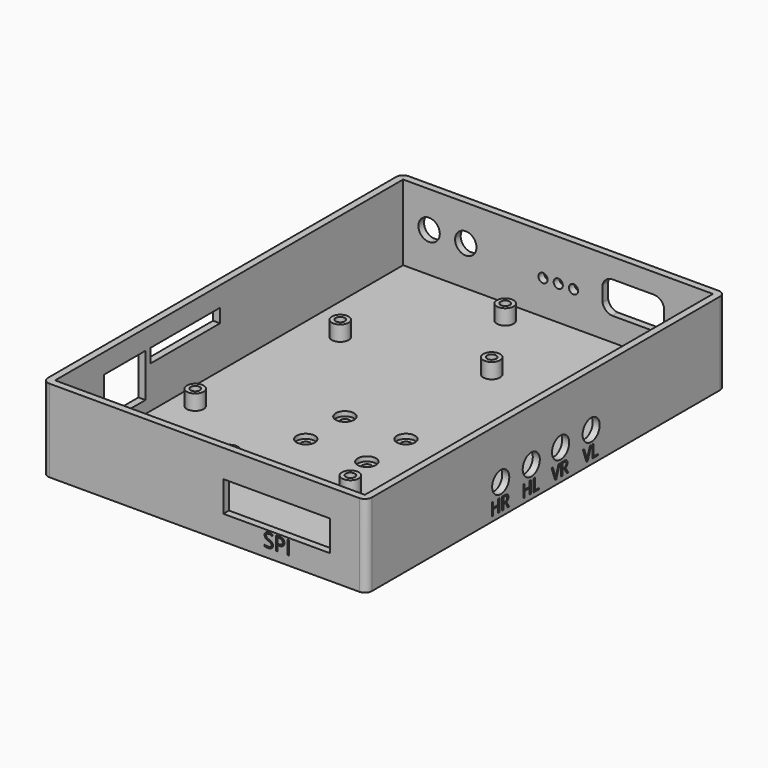
from build123d import *

# Parameters (mm, degrees)
F0_W            = 106
F0_H            = 147
F1_DEPTH        = 27
F2_T            = -2.3
F3_W            = 17
F3_H            = 14.2
F3_W_2          = 28.5
F3_H_2          = 4.5
F4_DEPTH        = 2.3
F5_R            = 2.3
F7_DEPTH        = 2.3
F9_DEPTH        = 2.3
F10_R           = 3.5
F10_R_2         = 1.5
F11_DEPTH       = 2.3
F12_TEXT_SIZE   = 5.6944444444
F13_DEPTH       = 1.0021
F14_TEXT_SIZE   = 6.25
F15_DEPTH       = 1
F16_TEXT_SIZE   = 4.2000262502
F16_TEXT_SIZE_2 = 6.8394336094
F16_TEXT_SIZE_3 = 6.6666666667
F16_TEXT_SIZE_4 = 6.25
F17_DEPTH       = 1
F18_DEPTH       = 1
F20_R           = 3
F20_R_2         = 1.5
F21_DEPTH       = 1.5
F22_DEPTH       = 2.3
F23_R           = 2.75
F24_DEPTH       = 5
F25_R           = 1.527073586
F26_DEPTH       = 2.5
F27_R           = 1.5414373887
F28_DEPTH       = 2.5
F29_R           = 1.5334502913
F30_DEPTH       = 2.5
F31_R           = 1.5249444559
F32_DEPTH       = 2.5
F33_R           = 1.5
F34_DEPTH       = 2.5
F35_R           = 1.5
F36_DEPTH       = 2.5
F37_R           = 1.5
F38_DEPTH       = 5
F39_R           = 1.5
F40_DEPTH       = 5
F41_R           = 1.5
F42_DEPTH       = 5
F43_R           = 1.5
F44_DEPTH       = 5
F45_R           = 1.5
F46_DEPTH       = 5


# Not quite as in the source:
# - Text() gives the source's letters only with a copy of the font that has no kerning and outlines rounded to 1/6400 em; it was checked with that copy


with BuildPart() as f1:
    # F0 (on Top) → F1 (new body)
    with BuildSketch(Plane.XY):
        with Locations((8.4141408205, 41.5227819189)):
            Rectangle(F0_W, F0_H)
    extrude(amount=F1_DEPTH)

    # F2
    f2_openings = [f1.faces().sort_by_distance(p)[0] for p in [
        (8.414141, 41.522782, 27),
    ]]
    offset(amount=F2_T, openings=f2_openings)

    # F3 (on face) → F4 (cut, through all)
    with BuildSketch(Plane(origin=(-44.5858591795, 0, 0), x_dir=(0, -1, 0), z_dir=(-1, 0, 0))):
        with Locations((1.1772180811, 13.4)):
            Rectangle(F3_W, F3_H)
        with Locations((-23.5727819189, 18.25)):
            Rectangle(F3_W_2, F3_H_2)
    extrude(amount=-F4_DEPTH, mode=Mode.SUBTRACT)

    # F5
    f5_edges = [f1.edges().sort_by_distance(p)[0] for p in [
        (-44.585859, -31.977218, 13.5),
        (61.414141, -31.977218, 13.5),
        (61.414141, 115.022782, 13.5),
        (-44.585859, 115.022782, 13.5),
    ]]
    fillet(f5_edges, radius=F5_R)

    # F6 (on face) → F7 (cut, through all)
    with BuildSketch(Plane.XZ.offset(31.9772180811)):
        Polygon((14.6141408205, 8), (23.1141408205, 8), (38.5841408205, 8), (49.6141408205, 8), (49.6141408205, 18), (14.6141408205, 18), align=None)
    extrude(amount=-F7_DEPTH, mode=Mode.SUBTRACT)

    # F8 (on face) → F9 (cut, through all)
    with BuildSketch(Plane.YZ.offset(61.4141408205)):
        with BuildLine():
            ThreePointArc((26.5227819189, 10), (23.0227819189, 13.5), (19.5227819189, 10))
            Line((19.5227819189, 10), (26.5227819189, 10))
        make_face()
        with BuildLine():
            ThreePointArc((63.5227819189, 10), (60.0227819189, 13.5), (56.5227819189, 10))
            Line((56.5227819189, 10), (63.5227819189, 10))
        make_face()
        with BuildLine():
            Line((63.5227819189, 10), (56.5227819189, 10))
            ThreePointArc((56.5227819189, 10), (60.0227819189, 6.5), (63.5227819189, 10))
        make_face()
        with BuildLine():
            ThreePointArc((51.0227819189, 10), (47.5227819189, 13.5), (44.0227819189, 10))
            Line((44.0227819189, 10), (51.0227819189, 10))
        make_face()
        with BuildLine():
            Line((51.0227819189, 10), (44.0227819189, 10))
            ThreePointArc((44.0227819189, 10), (47.5227819189, 6.5), (51.0227819189, 10))
        make_face()
        with BuildLine():
            ThreePointArc((39.0227819189, 10), (35.5227819189, 13.5), (32.0227819189, 10))
            Line((32.0227819189, 10), (35.5227819189, 10))
            Line((35.5227819189, 10), (39.0227819189, 10))
        make_face()
        with BuildLine():
            Line((35.5227819189, 10), (32.0227819189, 10))
            ThreePointArc((32.0227819189, 10), (35.5227819189, 6.5), (39.0227819189, 10))
            Line((39.0227819189, 10), (35.5227819189, 10))
        make_face()
        with BuildLine():
            Line((26.5227819189, 10), (19.5227819189, 10))
            ThreePointArc((19.5227819189, 10), (23.0227819189, 6.5), (26.5227819189, 10))
        make_face()
    extrude(amount=-F9_DEPTH, mode=Mode.SUBTRACT)

    # F10 (on face) → F11 (cut, through all)
    with BuildSketch(Plane(origin=(0, 115.0227819189, 0), x_dir=(-1, 0, 0), z_dir=(0, 1, 0))):
        with BuildLine():
            ThreePointArc((-43.1187852615, 12.6981928302), (-41.9758916203, 10.7926889432), (-39.9001278626, 10))
            Line((-39.9001278626, 10), (-26.2001278626, 10))
            ThreePointArc((-26.2001278626, 10), (-24.1282444641, 10.8027765078), (-22.994633107, 12.713817122))
            Line((-22.994633107, 12.713817122), (-22.9714840184, 17.8137645845))
            ThreePointArc((-22.9714840184, 17.8137645845), (-24.1214373626, 19.7150163417), (-26.2001269465, 20.5000007697))
            Line((-26.2001269465, 20.5000007697), (-39.9001269465, 20.5000007697))
            ThreePointArc((-39.9001269465, 20.5000007697), (-41.9749984238, 19.7049792034), (-43.1157495885, 17.7981919267))
            Line((-43.1157495885, 17.7981919267), (-43.1187852615, 12.6981928302))
        make_face()
        with Locations((21.7858591795, 15.25)):
            Circle(F10_R)
        with Locations((33.7858591795, 15.25)):
            Circle(F10_R)
        with Locations((-13.490966692, 13.5)):
            Circle(F10_R_2)
        with Locations((-8.490966692, 13.5)):
            Circle(F10_R_2)
        with Locations((-3.490966692, 13.5)):
            Circle(F10_R_2)
    extrude(amount=-F11_DEPTH, mode=Mode.SUBTRACT)

    # F12 (on face) → F13 (cut)
    with BuildSketch(Plane.YZ.offset(61.4141408205)):
        with Locations((18.8413870574, 1.527368344)):
            Text('HR', F12_TEXT_SIZE, font='Open Sans', text_align=(TextAlign.LEFT, TextAlign.BOTTOM))
        with Locations((31.723804778, 1.527368344)):
            Text('HL', F12_TEXT_SIZE, font='Open Sans', text_align=(TextAlign.LEFT, TextAlign.BOTTOM))
        with Locations((43.8213076026, 1.527368344)):
            Text('VR', F12_TEXT_SIZE, font='Open Sans', text_align=(TextAlign.LEFT, TextAlign.BOTTOM))
        with Locations((56.6572342636, 1.527368344)):
            Text('VL', F12_TEXT_SIZE, font='Open Sans', text_align=(TextAlign.LEFT, TextAlign.BOTTOM))
    extrude(amount=-F13_DEPTH, mode=Mode.SUBTRACT)

    # F14 (on face) → F15 (cut)
    with BuildSketch(Plane.XZ.offset(31.9772180811)):
        with Locations((27.7489064455, 2.9447209382)):
            Text('SPI', F14_TEXT_SIZE, font='Open Sans', text_align=(TextAlign.LEFT, TextAlign.BOTTOM))
    extrude(amount=-F15_DEPTH, mode=Mode.SUBTRACT)

    # F16 (on face) → F17 (cut)
    with BuildSketch(Plane(origin=(0, 115.0227819189, 0), x_dir=(-1, 0, 0), z_dir=(0, 1, 0))):
        with Locations((-53.0501269465, 21.3000007697)):
            Text('Can 120 OHM Inside', F16_TEXT_SIZE, font='Open Sans', text_align=(TextAlign.LEFT, TextAlign.BOTTOM))
        with Locations((19.7858591795, 6.8256078012)):
            Text('+', F16_TEXT_SIZE_2, font='Open Sans', text_align=(TextAlign.LEFT, TextAlign.BOTTOM))
        with Locations((32.6337758462, 6.95)):
            Text('-', F16_TEXT_SIZE_3, font='Open Sans', text_align=(TextAlign.LEFT, TextAlign.BOTTOM))
        with Locations((22.150116992, 18.7309935717)):
            Text('12V', F16_TEXT_SIZE_4, font='Open Sans', text_align=(TextAlign.LEFT, TextAlign.BOTTOM))
    extrude(amount=-F17_DEPTH, mode=Mode.SUBTRACT)

    # F16 (on face) → F18 (cut)
    with BuildSketch(Plane(origin=(0, 115.0227819189, 0), x_dir=(-1, 0, 0), z_dir=(0, 1, 0))):
        with Locations((-53.0501269465, 21.3000007697)):
            Text('Can 120 OHM Inside', F16_TEXT_SIZE, font='Open Sans', text_align=(TextAlign.LEFT, TextAlign.BOTTOM))
        with Locations((19.7858591795, 6.8256078012)):
            Text('+', F16_TEXT_SIZE_2, font='Open Sans', text_align=(TextAlign.LEFT, TextAlign.BOTTOM))
        with Locations((32.6337758462, 6.95)):
            Text('-', F16_TEXT_SIZE_3, font='Open Sans', text_align=(TextAlign.LEFT, TextAlign.BOTTOM))
        with Locations((22.150116992, 18.7309935717)):
            Text('12V', F16_TEXT_SIZE_4, font='Open Sans', text_align=(TextAlign.LEFT, TextAlign.BOTTOM))
    extrude(amount=-F18_DEPTH, mode=Mode.SUBTRACT)

    # F20 (on face) → F21 (cut)
    with BuildSketch(Plane.XY.offset(2.3)):
        with Locations((-1.5858591795, 38.0227819189)):
            Circle(F20_R)
        with Locations((-1.5858591795, 38.0227819189)):
            Circle(F20_R_2, mode=Mode.SUBTRACT)
        with BuildLine():
            ThreePointArc((21.4141408205, 38.0227819189), (18.4141408205, 41.0227819189), (15.4141408205, 38.0227819189))
            ThreePointArc((15.4141408205, 38.0227819189), (18.4141408205, 35.0227819189), (21.4141408205, 38.0227819189))
        make_face()
        with BuildLine():
            ThreePointArc((19.9141408205, 38.0227819189), (18.4141408205, 36.5227819189), (16.9141408205, 38.0227819189))
            ThreePointArc((16.9141408205, 38.0227819189), (18.4141408205, 39.5227819189), (19.9141408205, 38.0227819189))
        make_face(mode=Mode.SUBTRACT)
        with Locations((-1.5858591795, 22.0227819189)):
            Circle(F20_R)
        with Locations((-1.5858591795, 22.0227819189)):
            Circle(F20_R_2, mode=Mode.SUBTRACT)
        with Locations((18.4141408205, 22.0227819189)):
            Circle(F20_R)
        with Locations((18.4141408205, 22.0227819189)):
            Circle(F20_R_2, mode=Mode.SUBTRACT)
    extrude(amount=-F21_DEPTH, mode=Mode.SUBTRACT)

    # F22 (cut, through all): faces of the model
    f22_faces = [f1.faces().sort_by_distance(p)[0] for p in [
        (18.4141408205, 22.0227819189, 2.3),
        (-1.5858591795, 22.0227819189, 2.3),
        (-1.5858591795, 38.0227819189, 2.3),
        (18.4141408205, 38.0227819189, 2.3),
    ]]
    extrude(f22_faces, amount=-F22_DEPTH, mode=Mode.SUBTRACT)

    # F23 (on face) → F24 (join)
    with BuildSketch(Plane.XY.offset(2.3)):
        with Locations((53.7941408205, -24.4972180811)):
            Circle(F23_R)
        with Locations((-2.7234411854, 105.0427819189)):
            Circle(F23_R)
        with Locations((45.2525866657, 105.0427819189)):
            Circle(F23_R)
        with Locations((48.7141408205, 5.9827819189)):
            Circle(F23_R)
        with Locations((-30.0258591795, 71.6727819189)):
            Circle(F23_R)
        with Locations((39.2741345912, 79.6427819189)):
            Circle(F23_R)
        with Locations((-7.1658591795, -2.240232192)):
            Circle(F23_R)
        with Locations((25.8541408205, 5.9827819189)):
            Circle(F23_R)
        with Locations((13.1541408205, 79.6427819189)):
            Circle(F23_R)
        with Locations((-35.1058591795, 18.6827819189)):
            Circle(F23_R)
        with Locations((-35.1058591795, -24.4972180811)):
            Circle(F23_R)
    extrude(amount=F24_DEPTH)

    # F25 (on face) → F26 (cut, symmetric)
    with BuildSketch(Plane.XY.offset(7.3)):
        with Locations((-2.7234411854, 105.0427819189)):
            Circle(F25_R)
    extrude(amount=F26_DEPTH, both=True, mode=Mode.SUBTRACT)

    # F27 (on face) → F28 (cut, symmetric)
    with BuildSketch(Plane.XY.offset(7.3)):
        with Locations((45.2525866657, 105.0427819189)):
            Circle(F27_R)
    extrude(amount=F28_DEPTH, both=True, mode=Mode.SUBTRACT)

    # F29 (on face) → F30 (cut, symmetric)
    with BuildSketch(Plane.XY.offset(7.3)):
        with Locations((53.7941408205, -24.4972180811)):
            Circle(F29_R)
    extrude(amount=F30_DEPTH, both=True, mode=Mode.SUBTRACT)

    # F31 (on face) → F32 (cut, symmetric)
    with BuildSketch(Plane.XY.offset(7.3)):
        with Locations((48.7141408205, 5.9827819189)):
            Circle(F31_R)
    extrude(amount=F32_DEPTH, both=True, mode=Mode.SUBTRACT)

    # F33 (on face) → F34 (cut, symmetric)
    with BuildSketch(Plane.XY.offset(7.3)):
        with Locations((39.2741345912, 79.6427819189)):
            Circle(F33_R)
    extrude(amount=F34_DEPTH, both=True, mode=Mode.SUBTRACT)

    # F35 (on face) → F36 (cut, symmetric)
    with BuildSketch(Plane.XY.offset(7.3)):
        with Locations((-30.0258591795, 71.6727819189)):
            Circle(F35_R)
    extrude(amount=F36_DEPTH, both=True, mode=Mode.SUBTRACT)

    # F37 (on face) → F38 (cut)
    with BuildSketch(Plane.XY.offset(7.3)):
        with Locations((-7.1658591795, -2.240232192)):
            Circle(F37_R)
    extrude(amount=-F38_DEPTH, mode=Mode.SUBTRACT)

    # F39 (on face) → F40 (cut)
    with BuildSketch(Plane.XY.offset(7.3)):
        with Locations((25.8541408205, 5.9827819189)):
            Circle(F39_R)
    extrude(amount=-F40_DEPTH, mode=Mode.SUBTRACT)

    # F41 (on face) → F42 (cut)
    with BuildSketch(Plane.XY.offset(7.3)):
        with Locations((13.1541408205, 79.6427819189)):
            Circle(F41_R)
    extrude(amount=-F42_DEPTH, mode=Mode.SUBTRACT)

    # F43 (on face) → F44 (cut)
    with BuildSketch(Plane.XY.offset(7.3)):
        with Locations((-35.1058591795, 18.6827819189)):
            Circle(F43_R)
    extrude(amount=-F44_DEPTH, mode=Mode.SUBTRACT)

    # F45 (on face) → F46 (cut)
    with BuildSketch(Plane.XY.offset(7.3)):
        with Locations((-35.1058591795, -24.4972180811)):
            Circle(F45_R)
    extrude(amount=-F46_DEPTH, mode=Mode.SUBTRACT)


solid = f1.part
